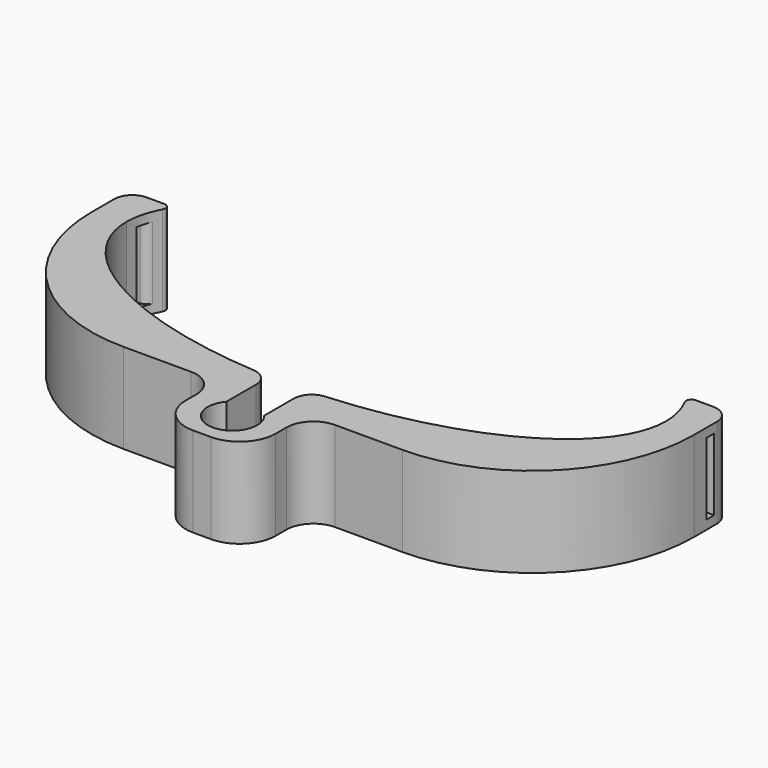
from build123d import *

# Parameters (mm, degrees)
F2_W      = 12.7
F2_H      = 10.795
F5_DEPTH  = 12.7
F0_W      = 85.09
F0_H      = 46.99
F7_DEPTH  = 12.7
F3_R      = 3.4925
F4_W      = 5.334
F4_H      = 12.7
F8_DEPTH  = 12.7
F10_DEPTH = 12.7
F12_R     = 3.81
F13_R     = 22.86
F14_R     = 5.08
F15_R     = 2.54
F16_R     = 0.762
F17_W     = 1.3
F17_H     = 10.16
F18_DEPTH = 88.9
F19_R     = 1.27


# Not quite as in the source:
# - a feature of the source that left no trace in its solid (it failed there, or was rolled back) is left out


with BuildPart() as f5:
    # F2 (on Top) → F5 (new body)
    with BuildSketch(Plane.XY):
        with Locations((0, -13.0144613445)):
            Rectangle(F2_W, F2_H)
    extrude(amount=F5_DEPTH)


with BuildPart() as f5b:
    # F0 (on Top) → F5, piece 2 (new body)
    with BuildSketch(Plane.XY):
        with Locations((0, 15.8780386555)):
            Rectangle(F0_W, F0_H)
    extrude(amount=F5_DEPTH)

    # F6: union F5
    add(f5.part)

    # F1 (on face) → F7 (cut)
    with BuildSketch(Plane.XY):
        with BuildLine():
            add(Edge.make_bspline(
                [(-38.1, 15.8780386555), (-38.1, -17.1175292287), (19.05, -0.6197452866), (76.2, 15.8780386555), (19.05, 32.3758225976), (-38.1, 48.8736065397), (-38.1, 15.8780386555)],
                knots=[0, 0, 0, 2.0943951024, 2.0943951024, 4.1887902048, 4.1887902048, 6.2831853072, 6.2831853072, 6.2831853072], degree=2, weights=[1, 0.5, 1, 0.5, 1, 0.5, 1]))
        make_face()
    extrude(amount=F7_DEPTH, mode=Mode.SUBTRACT)

    # F3 (on Top) + F4 (on Top) → F8 (cut)
    with BuildSketch(Plane.XY):
        with Locations((0, -13.0144613445)):
            Circle(F3_R)
    with BuildSketch(Plane.XY):
        with Locations((0, -6.6644613445)):
            Rectangle(F4_W, F4_H)
    extrude(amount=F8_DEPTH, mode=Mode.SUBTRACT)

    # F9 (on face) → F10 (cut)
    with BuildSketch(Plane.XY.offset(12.7)):
        Polygon((48.7572182757, 21.839483929), (48.7572182757, 42.4993435767), (-49.0327817243, 42.4993435767), (-49.0327817243, 21.839483929), (-42.545, 21.839483929), (-42.545, 39.3730386555), (42.545, 39.3730386555), (42.545, 21.839483929), align=None)
        with BuildLine():
            Line((36.1863880624, 21.839483929), (42.545, 21.839483929))
            Line((42.545, 21.839483929), (42.545, 39.3730386555))
            Line((42.545, 39.3730386555), (-42.545, 39.3730386555))
            Line((-42.545, 39.3730386555), (-42.545, 21.839483929))
            Line((-42.545, 21.839483929), (-36.1863880624, 21.839483929))
            add(Edge.make_bspline(
                [(36.1863880624, 21.839483929), (31.637806335, 28.7420359095), (19.05, 32.3758225976), (-21.5247671589, 44.0887489683), (-36.1863880624, 21.839483929)],
                knots=[3.4327056268, 3.4327056268, 3.4327056268, 4.1887902048, 4.1887902048, 5.9279520588, 5.9279520588, 5.9279520588], degree=2, weights=[0.7693199453, 0.819498103, 1, 0.5848056911, 0.8591566387]))
        make_face()
    extrude(amount=-F10_DEPTH, mode=Mode.SUBTRACT)

    # F12
    f12_edges = [f5b.edges().sort_by_distance(p)[0] for p in [
        (-6.35, -7.616961, 6.35),
        (6.35, -7.616961, 6.35),
    ]]
    fillet(f12_edges, radius=F12_R)

    # F13
    f13_edges = [f5b.edges().sort_by_distance(p)[0] for p in [
        (-42.545, -7.616961, 6.35),
        (42.545, -7.616961, 6.35),
    ]]
    fillet(f13_edges, radius=F13_R)

    # F14
    f14_edges = [f5b.edges().sort_by_distance(p)[0] for p in [
        (-6.35, -18.411961, 6.35),
        (6.35, -18.411961, 6.35),
    ]]
    fillet(f14_edges, radius=F14_R)

    # F15
    f15_edges = [f5b.edges().sort_by_distance(p)[0] for p in [
        (-42.545, 21.839484, 6.35),
        (42.545, 21.839484, 6.35),
        (2.667, -3.125232, 6.35),
        (-2.667, -3.125232, 6.35),
    ]]
    fillet(f15_edges, radius=F15_R)

    # F16
    f16_edges = [f5b.edges().sort_by_distance(p)[0] for p in [
        (-36.186388, 21.839484, 6.35),
        (36.186388, 21.839484, 6.35),
    ]]
    fillet(f16_edges, radius=F16_R)

    # F17 (on face) → F18 (cut)
    with BuildSketch(Plane(origin=(-42.545, 0, 0), x_dir=(0, -1, 0), z_dir=(-1, 0, 0))):
        with Locations((-18.1576684117, 6.35)):
            Rectangle(F17_W, F17_H)
    extrude(amount=-F18_DEPTH, mode=Mode.SUBTRACT)

    # F19
    f19_edges = [f5b.edges().sort_by_distance(p)[0] for p in [
        (37.646767, 18.807668, 6.35),
        (-37.646767, 18.807668, 6.35),
    ]]
    fillet(f19_edges, radius=F19_R)


solid = f5b.part
